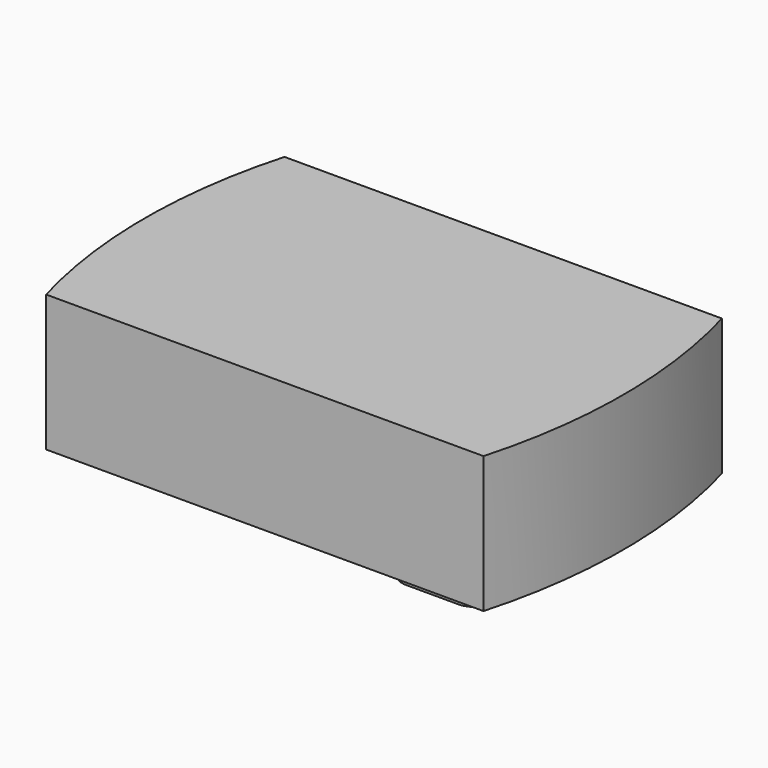
from build123d import *

# Parameters (mm, degrees)
F1_DEPTH     = 25
F2_W         = 42.6678306208
F2_H         = 26.6738910404
F3_DEPTH     = 3
F4_R         = 3
F5_DEPTH     = 1.5
F6_TEXT_SIZE = 20.0752823087
F7_DEPTH     = 2


# Not quite as in the source:
# - Text() gives the source's letters only with a copy of the font that has no kerning and outlines rounded to 1/6400 em; it was checked with that copy


with BuildPart() as f1:
    # F0 (on Top) → F1 (new body)
    with BuildSketch(Plane.XY):
        with BuildLine():
            Line((40.075, 27.3038461538), (-40.075, 27.3038461538))
            ThreePointArc((-40.075, 27.3038461538), (-43.8339153104, 0), (-40.075, -27.3038461538))
            Line((-40.075, -27.3038461538), (40.075, -27.3038461538))
            ThreePointArc((40.075, -27.3038461538), (43.8339153104, 0), (40.075, 27.3038461538))
        make_face()
    extrude(amount=F1_DEPTH)

    # F2 (on Top) → F3 (cut)
    with BuildSketch(Plane.XY):
        with Locations((0, 2.9283927666)):
            Rectangle(F2_W, F2_H)
    extrude(amount=F3_DEPTH, mode=Mode.SUBTRACT)

    # F4 (on Top) → F5 (join)
    with BuildSketch(Plane.XY):
        with Locations((-30.8802641788, -21.0485527536)):
            Circle(F4_R)
        with Locations((-19.8802641788, -21.0485527536)):
            Circle(F4_R)
        with Locations((-8.8802641788, -21.0485527536)):
            Circle(F4_R)
        with Locations((2.1197358212, -21.0485527536)):
            Circle(F4_R)
        with Locations((13.1197358212, -21.0485527536)):
            Circle(F4_R)
        with BuildLine():
            ThreePointArc((24.6570557356, -17.8247001022), (20.7339162007, -21.7478396371), (24.6570557356, -25.670979172))
            Line((24.6570557356, -25.670979172), (34.1155827045, -25.670979172))
            ThreePointArc((34.1155827045, -25.670979172), (38.0982689183, -21.8977586736), (34.5455147326, -17.7172180265))
            Line((34.5455147326, -17.7172180265), (24.6570557356, -17.8247001022))
        make_face()
    extrude(amount=-F5_DEPTH)

    # F6 (on face) → F7 (join)
    with BuildSketch(Plane(origin=(0, 0, 3), x_dir=(1, 0, 0), z_dir=(0, 0, -1))):
        with Locations((-20, -8.2420011592)):
            Text('90:9', F6_TEXT_SIZE, font='Open Sans', text_align=(TextAlign.LEFT, TextAlign.BOTTOM))
    extrude(amount=F7_DEPTH)


solid = f1.part
